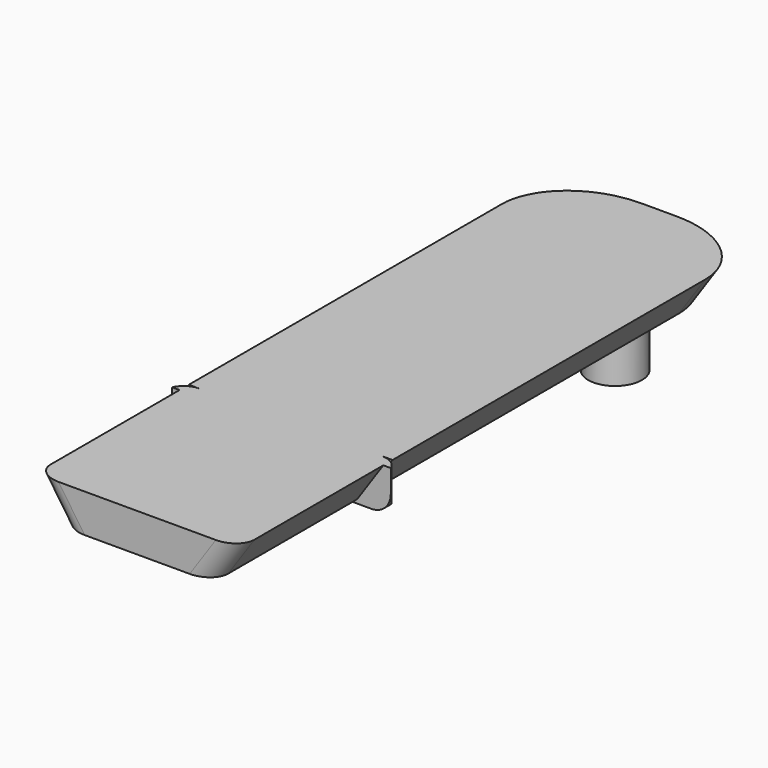
from build123d import *

# Parameters (mm, degrees)
F1_DEPTH    = 50
F2_DEPTH    = 3
F3_T1_DEPTH = 28
F3_T3_DEPTH = 33.9128784748
F4_DEPTH    = 120
F5_T1_DEPTH = 102.6362149123
F5_T3_DEPTH = 102.6362149123
F6_R        = 11
F7_DEPTH    = 4
F8_R        = 7
F9_DEPTH    = 17
F10_R       = 5


# Not quite as in the source:
# - a fillet or chamfer that OpenCascade refuses, or shapes differently, is made with other operations: its cross-section is extruded or revolved along the edge and cut away or added


with BuildPart() as f1:
    # F0 (on Front) → F1 (new body)
    with BuildSketch(Plane.XZ):
        Polygon((26.5539305929, 3.625), (-26.5539305929, 3.625), (-19.7357487747, -6.375), (19.7357487747, -6.375), align=None)
    extrude(amount=F1_DEPTH)

    # F0 (on Front) → F2 (join)
    with BuildSketch(Plane.XZ):
        Polygon((20, -6.875), (-20, -6.875), (-27.1590909091, 3.625), (-27.5, 3.625), (-28.5, 3.625), (-28.5, -7.375), (28.5, -7.375), (28.5, 3.625), (27.5, 3.625), (27.1590909091, 3.625), align=None)
        Polygon((26.5539305929, 3.625), (-26.5539305929, 3.625), (-19.7357487747, -6.375), (19.7357487747, -6.375), align=None)
        Polygon((-27.1590909091, 3.625), (-20, -6.875), (20, -6.875), (27.1590909091, 3.625), (26.5539305929, 3.625), (19.7357487747, -6.375), (-19.7357487747, -6.375), (-26.5539305929, 3.625), align=None)
    extrude(amount=F2_DEPTH)

    # F3: fillet of radius 5 on 4 edges, made by hand

    # F3_s2 → F3_t1 (cut)
    with BuildSketch(Plane.XZ.offset(-12.5)):
        with BuildLine():
            ThreePointArc((28.5, -2.375), (27.0355339059, -5.9105339059), (23.5, -7.375))
            Line((23.5, -7.375), (28.5, -7.375))
            Line((28.5, -7.375), (28.5, -2.375))
        make_face()
        with BuildLine():
            ThreePointArc((-23.5, -7.375), (-27.0355339059, -5.9105339059), (-28.5, -2.375))
            Line((-28.5, -2.375), (-28.5, -7.375))
            Line((-28.5, -7.375), (-23.5, -7.375))
        make_face()
    extrude(amount=F3_T1_DEPTH, mode=Mode.SUBTRACT)

    # F3_s4 → F3_t3 (cut)
    with BuildSketch(Plane.XY.offset(-18.8314392374)):
        with BuildLine():
            ThreePointArc((23.917424305, 0), (26.6560370926, -0.8166998673), (28.5, -3))
            Line((28.5, -3), (28.5, 0))
            Line((28.5, 0), (23.917424305, 0))
        make_face()
        with BuildLine():
            ThreePointArc((-23.917424305, 0), (-26.6560370926, -0.8166998673), (-28.5, -3))
            Line((-28.5, -3), (-28.5, 0))
            Line((-28.5, 0), (-23.917424305, 0))
        make_face()
    extrude(amount=F3_T3_DEPTH, mode=Mode.SUBTRACT)

    # F0 (on Front) → F4 (join)
    with BuildSketch(Plane.XZ):
        Polygon((26.5539305929, 3.625), (-26.5539305929, 3.625), (-19.7357487747, -6.375), (19.7357487747, -6.375), align=None)
    extrude(amount=-F4_DEPTH)

    # F5: fillet of radius 18.1066017178 on 2 edges, made by hand

    # F5_s2 → F5_t1 (cut)
    with BuildSketch(Plane(origin=(-22.2043882639, 0, -32.5664361204), x_dir=(0, 1, 0), z_dir=(0.5633368246, 0, 0.8262273428))):
        with BuildLine():
            ThreePointArc((101.8933982822, -19.8974875256), (114.6966991411, -14.5941866667), (120, -1.7908858078))
            Line((120, -1.7908858078), (120, -19.8974875256))
            Line((120, -19.8974875256), (101.8933982822, -19.8974875256))
        make_face()
    extrude(amount=F5_T1_DEPTH, mode=Mode.SUBTRACT)

    # F5_s4 → F5_t3 (cut)
    with BuildSketch(Plane(origin=(-35.614371138, 0, 52.2344110024), x_dir=(0, 1, 0), z_dir=(0.5633368246, 0, -0.8262273428))):
        with BuildLine():
            ThreePointArc((101.8933982822, -19.8974875256), (114.6966991411, -14.5941866667), (120, -1.7908858078))
            Line((120, -1.7908858078), (120, -19.8974875256))
            Line((120, -19.8974875256), (101.8933982822, -19.8974875256))
        make_face()
    extrude(amount=F5_T3_DEPTH, mode=Mode.SUBTRACT)

    # F6 (on face) → F7 (join)
    with BuildSketch(Plane(origin=(0, 0, -6.375), x_dir=(1, 0, 0), z_dir=(0, 0, -1))):
        with Locations((0, -105.7220622897)):
            Circle(F6_R)
    extrude(amount=F7_DEPTH)

    # F8 (on face) → F9 (join)
    with BuildSketch(Plane(origin=(0, 0, -10.375), x_dir=(1, 0, 0), z_dir=(0, 0, -1))):
        with Locations((0, -105.7220622897)):
            Circle(F8_R)
    extrude(amount=F9_DEPTH)

    # F10
    f10_edges = [f1.edges().sort_by_distance(p)[0] for p in [
        (23.14484, -50, -1.375),
        (-23.14484, -50, -1.375),
    ]]
    fillet(f10_edges, radius=F10_R)


solid = f1.part
